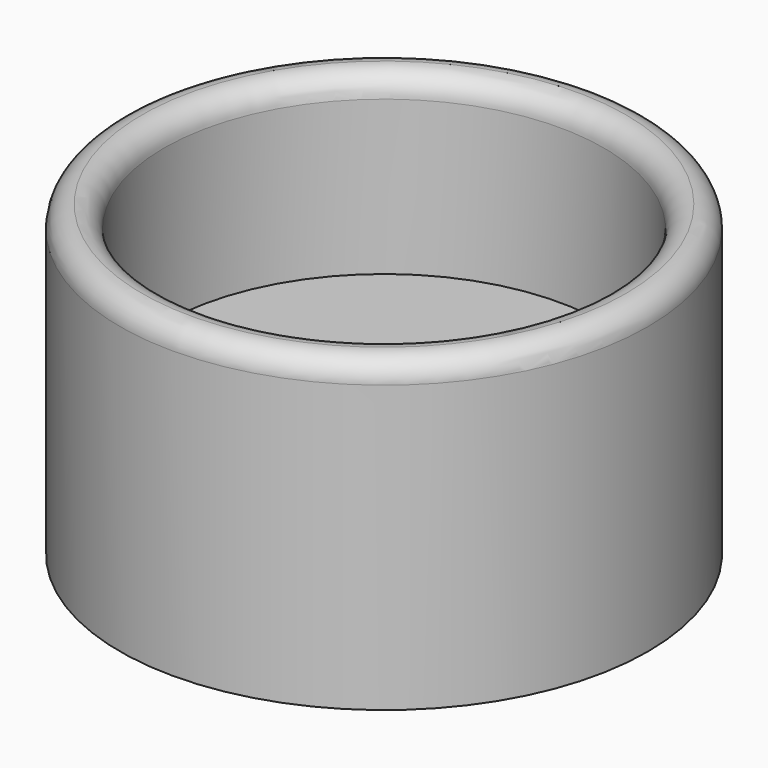
from build123d import *

# Parameters (mm, degrees)
F0_R     = 6
F0_R_2   = 5
F1_DEPTH = 7
F2_DEPTH = 3
F3_R     = 0.49999


# Not quite as in the source:
# - a fillet or chamfer is up to 0.001 mm smaller than in the source, because OpenCascade refuses the exact size


with BuildPart() as f1:
    # F0 (on Top) → F1 (new body)
    with BuildSketch(Plane.XY):
        Circle(F0_R)
        Circle(F0_R_2, mode=Mode.SUBTRACT)
    extrude(amount=F1_DEPTH)

    # F0 (on Top) → F2 (join)
    with BuildSketch(Plane.XY):
        Circle(F0_R_2)
    extrude(amount=F2_DEPTH)

    # F3 (radius 0.5 in the source; OpenCascade refuses exactly that, so slightly less here)
    f3_edges = [f1.edges().sort_by_distance(p)[0] for p in [
        (-6, 0, 7),
        (-5, 0, 7),
    ]]
    fillet(f3_edges, radius=F3_R)


solid = f1.part
